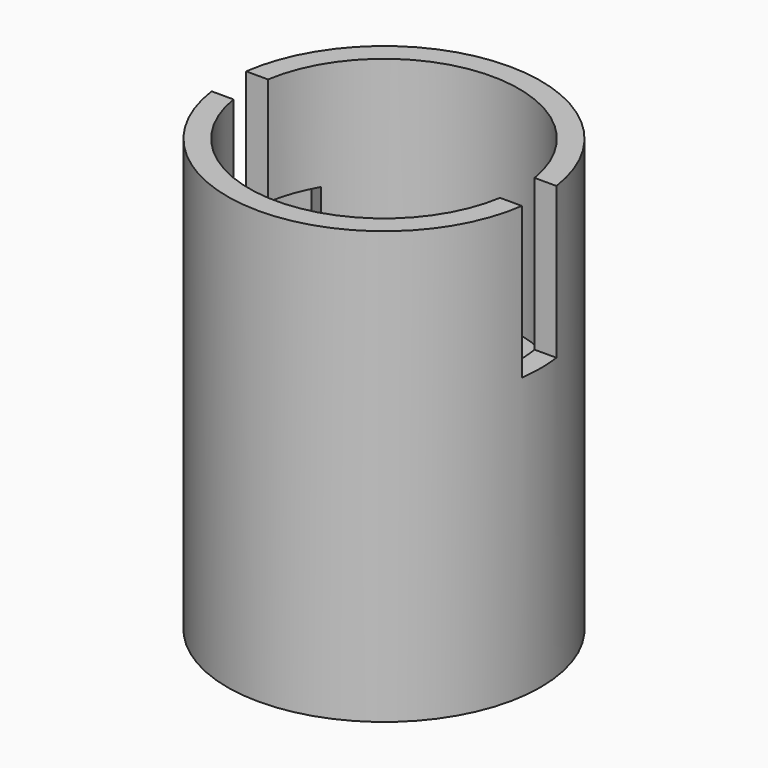
from build123d import *

# Parameters (mm, degrees)
F4_DEPTH        = 25.4
F5_W            = 12.7
F5_H            = 5.08
F6_ANGLE        = 30
F6_COPIES_COUNT = 2


# Not quite as in the source:
# - a pattern or mirror of a feature is missing from the dataset's text; its kind, count and spacing are read off the source's solid


with BuildPart() as f2:
    # F0 (on Front) → F2 (revolve)
    with BuildSketch(Plane.XZ):
        Polygon((18.415, 63.2877647877), (15.875, 63.2877647877), (15.875, 37.8877647877), (12.7, 37.8877647877), (12.7, 12.4877647877), (18.415, 12.4877647877), align=None)
    revolve(axis=Axis((0, 0, -2.1974854171), (0, 0, -1)))

    # F3 (on Right) → F4 (cut, symmetric)
    with BuildSketch(Plane.YZ):
        Polygon((0, 63.2877647877), (-2.54, 63.2877647877), (-2.54, 45.5077647877), (0, 45.5077647877), (2.54, 45.5077647877), (2.54, 63.2877647877), align=None)
    extrude(amount=F4_DEPTH, both=True, mode=Mode.SUBTRACT)

    # F5 (on Front) → F6 (revolve, cut)
    with BuildSketch(Plane.XZ):
        with Locations((12.0015, 48.0477647877)):
            Rectangle(F5_W, F5_H)
    f6 = revolve(axis=Axis((0, 0, 12.4877647877), (0, 0, -1)), revolution_arc=F6_ANGLE, mode=Mode.SUBTRACT)

    # F6_copies: F6 ×2 about axis
    f6_copies_axis = Axis((0, 0, 0), (0, 0, 1))
    for i in range(1, F6_COPIES_COUNT):
        add(f6.rotate(f6_copies_axis, i * 360 / F6_COPIES_COUNT), mode=Mode.SUBTRACT)


solid = f2.part
